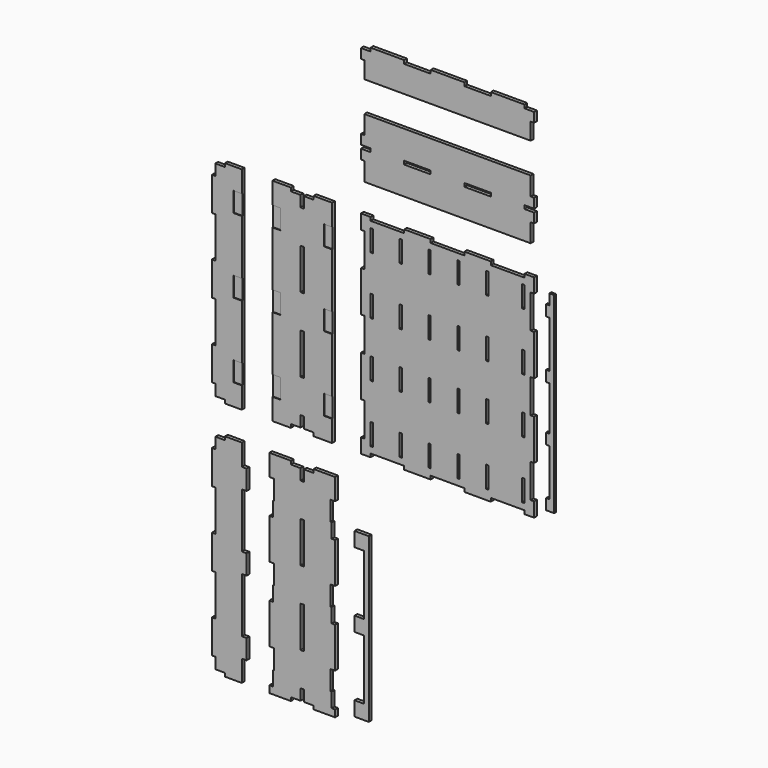
from build123d import *

# Parameters (mm, degrees)
F1_W     = 139.7
F1_H     = 18.034
F1_W_2   = 18.034
F1_H_2   = 50.8
F2_DEPTH = 18.034
F1_W_3   = 12.192
F1_H_3   = 113.5253
F1_H_4   = 215.9
F1_W_4   = 49.784
F1_H_5   = 76.2
F1_W_5   = 25.4
F1_H_6   = 104.14
F1_H_7   = 56.76265
F3_DEPTH = 12.192
F1_W_6   = 43.7134
F4_DEPTH = 14.7574


# Not quite as in the source:
# - a variable given as a bare number and used for a length is read in inches; the dataset says mm whatever the document's units were
# - a feature names something its author has since deleted; it is built from what else it names


with BuildPart() as f2:
    # F1 (on Front) → F2 (new body)
    with BuildSketch(Plane.XZ):
        Polygon((439.166, 1026.668), (-439.166, 1026.668), (-439.166, 928.751), (-439.166, 877.951), (-406.4, 877.951), (-406.4, 859.917), (-439.166, 859.917), (-439.166, 809.117), (-439.166, 711.2), (439.166, 711.2), (439.166, 809.117), (439.166, 859.917), (406.4, 859.917), (406.4, 877.951), (439.166, 877.951), (439.166, 928.751), align=None)
        with Locations((-158.75, 868.934)):
            Rectangle(F1_W, F1_H, mode=Mode.SUBTRACT)
        with Locations((158.75, 868.934)):
            Rectangle(F1_W, F1_H, mode=Mode.SUBTRACT)
        with Locations((-448.183, 903.351)):
            Rectangle(F1_W_2, F1_H_2)
        with Locations((-448.183, 834.517)):
            Rectangle(F1_W_2, F1_H_2)
        with Locations((448.183, 903.351)):
            Rectangle(F1_W_2, F1_H_2)
        with Locations((448.183, 834.517)):
            Rectangle(F1_W_2, F1_H_2)
    extrude(amount=F2_DEPTH)


with BuildPart() as f2b:
    # F1 (on Front) → F2, piece 2 (new body)
    with BuildSketch(Plane.XZ):
        Polygon((-406.4, 558.8), (-457.2, 558.8), (-457.2, 482.6), (-439.166, 482.6), (-439.166, 304.8), (-457.2, 304.8), (-457.2, 88.9), (-439.166, 88.9), (-439.166, -88.9), (-457.2, -88.9), (-457.2, -304.8), (-439.166, -304.8), (-439.166, -482.6), (-457.2, -482.6), (-457.2, -558.8), (-406.4, -558.8), (-406.4, -540.766), (-228.6, -540.766), (-228.6, -558.8), (-88.9, -558.8), (-88.9, -540.766), (88.9, -540.766), (88.9, -558.8), (228.6, -558.8), (228.6, -540.766), (406.4, -540.766), (406.4, -558.8), (457.2, -558.8), (457.2, -482.6), (439.166, -482.6), (439.166, -304.8), (457.2, -304.8), (457.2, -88.9), (439.166, -88.9), (439.166, 88.9), (457.2, 88.9), (457.2, 304.8), (439.166, 304.8), (439.166, 482.6), (457.2, 482.6), (457.2, 558.8), (406.4, 558.8), (406.4, 540.766), (228.6, 540.766), (228.6, 558.8), (88.9, 558.8), (88.9, 540.766), (-88.9, 540.766), (-88.9, 558.8), (-228.6, 558.8), (-228.6, 540.766), (-406.4, 540.766), align=None)
        with Locations((-399.5293, -450.46265)):
            Rectangle(F1_W_3, F1_H_3, mode=Mode.SUBTRACT)
        with Locations((-247.1293, -450.46265)):
            Rectangle(F1_W_3, F1_H_3, mode=Mode.SUBTRACT)
        with Locations((-94.7293, -450.46265)):
            Rectangle(F1_W_3, F1_H_3, mode=Mode.SUBTRACT)
        with Locations((57.6707, -450.46265)):
            Rectangle(F1_W_3, F1_H_3, mode=Mode.SUBTRACT)
        with Locations((210.0707, -450.46265)):
            Rectangle(F1_W_3, F1_H_3, mode=Mode.SUBTRACT)
        with Locations((399.5293, -450.46265)):
            Rectangle(F1_W_3, F1_H_3, mode=Mode.SUBTRACT)
        with Locations((-399.5293, -145.66265)):
            Rectangle(F1_W_3, F1_H_3, mode=Mode.SUBTRACT)
        with Locations((-399.5293, 145.66265)):
            Rectangle(F1_W_3, F1_H_3, mode=Mode.SUBTRACT)
        with Locations((-399.5293, 450.46265)):
            Rectangle(F1_W_3, F1_H_3, mode=Mode.SUBTRACT)
        with Locations((-247.1293, -145.66265)):
            Rectangle(F1_W_3, F1_H_3, mode=Mode.SUBTRACT)
        with Locations((-247.1293, 145.66265)):
            Rectangle(F1_W_3, F1_H_3, mode=Mode.SUBTRACT)
        with Locations((-94.7293, -145.66265)):
            Rectangle(F1_W_3, F1_H_3, mode=Mode.SUBTRACT)
        with Locations((57.6707, -145.66265)):
            Rectangle(F1_W_3, F1_H_3, mode=Mode.SUBTRACT)
        with Locations((-94.7293, 145.66265)):
            Rectangle(F1_W_3, F1_H_3, mode=Mode.SUBTRACT)
        with Locations((57.6707, 145.66265)):
            Rectangle(F1_W_3, F1_H_3, mode=Mode.SUBTRACT)
        with Locations((-247.1293, 450.46265)):
            Rectangle(F1_W_3, F1_H_3, mode=Mode.SUBTRACT)
        with Locations((-94.7293, 450.46265)):
            Rectangle(F1_W_3, F1_H_3, mode=Mode.SUBTRACT)
        with Locations((57.6707, 450.46265)):
            Rectangle(F1_W_3, F1_H_3, mode=Mode.SUBTRACT)
        with Locations((210.0707, -145.66265)):
            Rectangle(F1_W_3, F1_H_3, mode=Mode.SUBTRACT)
        with Locations((210.0707, 145.66265)):
            Rectangle(F1_W_3, F1_H_3, mode=Mode.SUBTRACT)
        with Locations((399.5293, -145.66265)):
            Rectangle(F1_W_3, F1_H_3, mode=Mode.SUBTRACT)
        with Locations((399.5293, 145.66265)):
            Rectangle(F1_W_3, F1_H_3, mode=Mode.SUBTRACT)
        with Locations((210.0707, 450.46265)):
            Rectangle(F1_W_3, F1_H_3, mode=Mode.SUBTRACT)
        with Locations((399.5293, 450.46265)):
            Rectangle(F1_W_3, F1_H_3, mode=Mode.SUBTRACT)
    extrude(amount=F2_DEPTH)


with BuildPart() as f2c:
    # F1 (on Front) → F2, piece 3 (new body)
    with BuildSketch(Plane.XZ):
        Polygon((-707.517, -558.8), (-609.6, -558.8), (-609.6, -445.77), (-653.3134, -445.77), (-653.3134, -341.63), (-609.6, -341.63), (-609.6, -52.07), (-653.3134, -52.07), (-653.3134, 52.07), (-609.6, 52.07), (-609.6, 341.63), (-653.3134, 341.63), (-653.3134, 445.77), (-609.6, 445.77), (-609.6, 558.8), (-707.517, 558.8), (-707.517, 540.766), (-758.317, 540.766), (-758.317, 482.6), (-776.351, 482.6), (-776.351, 540.766), (-827.151, 540.766), (-827.151, 558.8), (-925.068, 558.8), (-925.068, 445.77), (-881.3546, 445.77), (-881.3546, 341.63), (-925.068, 341.63), (-925.068, 52.07), (-881.3546, 52.07), (-881.3546, -52.07), (-925.068, -52.07), (-925.068, -341.63), (-881.3546, -341.63), (-881.3546, -445.77), (-925.068, -445.77), (-925.068, -558.8), (-827.151, -558.8), (-827.151, -540.766), (-776.351, -540.766), (-776.351, -482.6), (-758.317, -482.6), (-758.317, -540.766), (-707.517, -540.766), align=None)
        with Locations((-767.334, -196.85)):
            Rectangle(F1_W_2, F1_H_4, mode=Mode.SUBTRACT)
        with Locations((-767.334, 196.85)):
            Rectangle(F1_W_2, F1_H_4, mode=Mode.SUBTRACT)
    extrude(amount=F2_DEPTH)

    # F1 (on Front) → F4 (join)
    with BuildSketch(Plane.XZ):
        with Locations((-903.2113, 393.7)):
            Rectangle(F1_W_6, F1_H_6)
        with Locations((-631.4567, 393.7)):
            Rectangle(F1_W_6, F1_H_6)
        with Locations((-631.4567, 0)):
            Rectangle(F1_W_6, F1_H_6)
        with Locations((-903.2113, 0)):
            Rectangle(F1_W_6, F1_H_6)
        with Locations((-903.2113, -393.7)):
            Rectangle(F1_W_6, F1_H_6)
        with Locations((-631.4567, -393.7)):
            Rectangle(F1_W_6, F1_H_6)
    extrude(amount=F4_DEPTH)


with BuildPart() as f2d:
    # F1 (on Front) → F2, piece 4 (new body)
    with BuildSketch(Plane.XZ):
        with Locations((448.183, 1302.385)):
            Rectangle(F1_W_2, F1_H_2)
        with Locations((-448.183, 1302.385)):
            Rectangle(F1_W_2, F1_H_2)
        Polygon((228.6, 1345.819), (228.6, 1327.785), (88.9, 1327.785), (88.9, 1345.819), (-88.9, 1345.819), (-88.9, 1327.785), (-228.6, 1327.785), (-228.6, 1345.819), (-406.4, 1345.819), (-406.4, 1327.785), (-439.166, 1327.785), (-439.166, 1276.985), (-439.166, 1188.085), (439.166, 1188.085), (439.166, 1276.985), (439.166, 1327.785), (406.4, 1327.785), (406.4, 1345.819), align=None)
    extrude(amount=F2_DEPTH)


with BuildPart() as f2e:
    # F1 (on Front) → F2, piece 5 (new body)
    with BuildSketch(Plane.XZ):
        Polygon((-827.151, -711.2), (-940.943, -711.2), (-940.943, -824.23), (-915.543, -824.23), (-915.543, -928.37), (-922.909, -928.37), (-922.909, -1004.57), (-940.943, -1004.57), (-940.943, -1217.93), (-915.543, -1217.93), (-915.543, -1322.07), (-922.909, -1322.07), (-922.909, -1398.27), (-940.943, -1398.27), (-940.943, -1611.63), (-915.543, -1611.63), (-915.543, -1715.77), (-922.909, -1715.77), (-922.909, -1791.97), (-940.943, -1791.97), (-940.943, -1828.8), (-827.151, -1828.8), (-827.151, -1810.766), (-776.351, -1810.766), (-776.351, -1752.6), (-758.317, -1752.6), (-758.317, -1810.766), (-707.517, -1810.766), (-707.517, -1828.8), (-593.725, -1828.8), (-593.725, -1791.97), (-611.759, -1791.97), (-611.759, -1715.77), (-619.125, -1715.77), (-619.125, -1611.63), (-593.725, -1611.63), (-593.725, -1398.27), (-611.759, -1398.27), (-611.759, -1322.07), (-619.125, -1322.07), (-619.125, -1217.93), (-593.725, -1217.93), (-593.725, -1004.57), (-611.759, -1004.57), (-611.759, -928.37), (-619.125, -928.37), (-619.125, -824.23), (-593.725, -824.23), (-593.725, -711.2), (-707.517, -711.2), (-707.517, -729.234), (-758.317, -729.234), (-758.317, -787.4), (-776.351, -787.4), (-776.351, -729.234), (-827.151, -729.234), align=None)
        with Locations((-767.334, -1466.85)):
            Rectangle(F1_W_2, F1_H_4, mode=Mode.SUBTRACT)
        with Locations((-767.334, -1073.15)):
            Rectangle(F1_W_2, F1_H_4, mode=Mode.SUBTRACT)
    extrude(amount=F2_DEPTH)


with BuildPart() as f2f:
    # F1 (on Front) → F2, piece 6 (new body)
    with BuildSketch(Plane.XZ):
        with Locations((-466.217, -1360.17)):
            Rectangle(F1_W_4, F1_H_5)
        with Locations((-466.217, -1753.87)):
            Rectangle(F1_W_4, F1_H_5)
        Polygon((-415.925, -928.37), (-441.325, -928.37), (-441.325, -1004.57), (-441.325, -1322.07), (-441.325, -1398.27), (-441.325, -1715.77), (-441.325, -1791.97), (-415.925, -1791.97), align=None)
        with Locations((-466.217, -966.47)):
            Rectangle(F1_W_4, F1_H_5)
    extrude(amount=F2_DEPTH)


with BuildPart() as f2g:
    # F1 (on Front) → F2, piece 7 (new body)
    with BuildSketch(Plane.XZ):
        Polygon((-1175.385, 540.766), (-1226.185, 540.766), (-1226.185, 482.6), (-1244.219, 482.6), (-1244.219, 304.8), (-1226.185, 304.8), (-1226.185, 88.9), (-1244.219, 88.9), (-1244.219, -88.9), (-1226.185, -88.9), (-1226.185, -304.8), (-1244.219, -304.8), (-1244.219, -482.6), (-1226.185, -482.6), (-1226.185, -540.766), (-1175.385, -540.766), (-1175.385, -558.8), (-1086.485, -558.8), (-1086.485, -445.77), (-1130.1984, -445.77), (-1130.1984, -341.63), (-1086.485, -341.63), (-1086.485, -52.07), (-1130.1984, -52.07), (-1130.1984, 52.07), (-1086.485, 52.07), (-1086.485, 341.63), (-1130.1984, 341.63), (-1130.1984, 445.77), (-1086.485, 445.77), (-1086.485, 558.8), (-1175.385, 558.8), align=None)
    extrude(amount=F2_DEPTH)

    # F1 (on Front) → F4, piece 2 (join)
    with BuildSketch(Plane.XZ):
        with Locations((-1108.3417, -393.7)):
            Rectangle(F1_W_6, F1_H_6)
        with Locations((-1108.3417, 0)):
            Rectangle(F1_W_6, F1_H_6)
        with Locations((-1108.3417, 393.7)):
            Rectangle(F1_W_6, F1_H_6)
    extrude(amount=F4_DEPTH)


with BuildPart() as f2h:
    # F1 (on Front) → F2, piece 8 (new body)
    with BuildSketch(Plane.XZ):
        with Locations((-1073.785, -876.3)):
            Rectangle(F1_W_5, F1_H_6)
        with Locations((-1073.785, -1663.7)):
            Rectangle(F1_W_5, F1_H_6)
        with Locations((-1073.785, -1270)):
            Rectangle(F1_W_5, F1_H_6)
        Polygon((-1175.385, -729.234), (-1226.185, -729.234), (-1226.185, -787.4), (-1244.219, -787.4), (-1244.219, -965.2), (-1226.185, -965.2), (-1226.185, -1181.1), (-1244.219, -1181.1), (-1244.219, -1358.9), (-1226.185, -1358.9), (-1226.185, -1574.8), (-1244.219, -1574.8), (-1244.219, -1752.6), (-1226.185, -1752.6), (-1226.185, -1810.766), (-1175.385, -1810.766), (-1175.385, -1828.8), (-1086.485, -1828.8), (-1086.485, -1715.77), (-1086.485, -1611.63), (-1086.485, -1322.07), (-1086.485, -1217.93), (-1086.485, -928.37), (-1086.485, -824.23), (-1086.485, -711.2), (-1175.385, -711.2), align=None)
    extrude(amount=F2_DEPTH)


with BuildPart() as f3:
    # F1 (on Front) → F3 (new body)
    with BuildSketch(Plane.XZ):
        Polygon((558.8, 507.2253), (533.4, 507.2253), (533.4, 450.46265), (533.4, 393.7), (533.4, 145.66265), (533.4, 88.9), (533.4, -145.66265), (533.4, -202.4253), (533.4, -450.46265), (533.4, -507.2253), (558.8, -507.2253), align=None)
        with Locations((524.383, 422.081325)):
            Rectangle(F1_W_2, F1_H_7)
        with Locations((524.383, 117.281325)):
            Rectangle(F1_W_2, F1_H_7)
        with Locations((524.383, -174.043975)):
            Rectangle(F1_W_2, F1_H_7)
        with Locations((524.383, -478.843975)):
            Rectangle(F1_W_2, F1_H_7)
    extrude(amount=F3_DEPTH)


solid = Compound([f2.part, f2b.part, f2c.part, f2d.part, f2e.part, f2f.part, f2g.part, f2h.part, f3.part])
